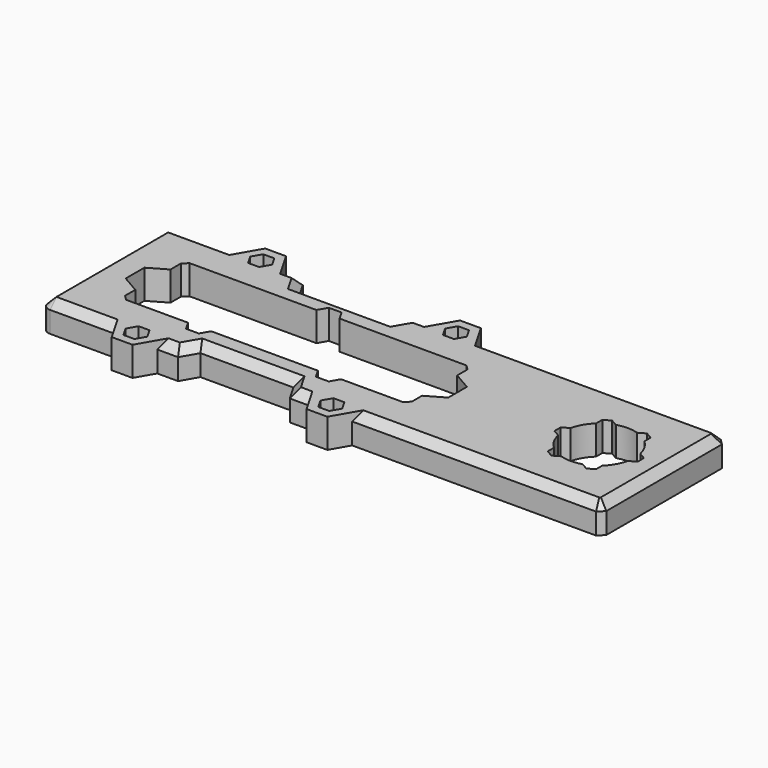
from build123d import *

# Parameters (mm, degrees)
F1_DEPTH      = 36.5
F2_SIZE       = 1.5
F4_DEPTH      = 75
F6_DEPTH      = 4.5
F8_DEPTH      = 4
F9_R          = 2.125
F10_DEPTH     = 4
F12_DEPTH     = 4
F13_R         = 2.125
F14_DEPTH     = 4
F15_R         = 2.125
F16_DEPTH     = 4
F18_DEPTH     = 32.75
F20_DEPTH     = 10
F21_R         = 2.125
F22_DEPTH     = 2
F23_W         = 33.9925625842
F23_H         = 3.75
F24_DEPTH     = 98.9435625842
F26_DEPTH     = 99
F27_T1_DEPTH  = 32.9343170514
F27_T3_DEPTH  = 25.8411991172
F28_T4_ANGLE  = 218.6312749598
F28_S5_R      = 11
F28_T6_DEPTH  = 16
F29_R         = 12.225
F29_R_2       = 4
F30_DEPTH     = 10
F31_T2_ANGLE  = 144.1325719132
F33_R         = 25
F34_DEPTH     = 25
F36_DEPTH     = 56.751
F37_T1_DEPTH  = 60.3629835333
F37_T3_DEPTH  = 29.9319647398
F37_T5_DEPTH  = 22.2894021556
F37_T7_DEPTH  = 111.8537479813
F37_T9_DEPTH  = 65.7902583728
F37_T11_DEPTH = 111.8554017465
F37_T13_DEPTH = 22.1084149398
F37_T15_DEPTH = 60.0584149398
F37_T17_DEPTH = 29.750977524
F40_DEPTH     = 56.751
F41_SIZE      = 1.5
F44_DEPTH     = 4
F45_R         = 2.125
F46_DEPTH     = 25
F47_R         = 2.125
F48_DEPTH     = 5
F50_DEPTH     = 4
F51_W         = 107.4425625842
F51_H         = 48
F52_DEPTH     = 47.751
F53_W         = 5
F53_H         = 48
F54_DEPTH     = 9
F55_R         = 2.5
F56_W         = 60
F56_H         = 48
F57_DEPTH     = 9
F58_SIZE      = 1.75
F59_W         = 4
F59_H         = 5.835
F60_DEPTH     = 9
F61_SIZE      = 2.49999


# Not quite as in the source:
# - a fillet or chamfer that OpenCascade refuses, or shapes differently, is made with other operations: its cross-section is extruded or revolved along the edge and cut away or added
# - a fillet or chamfer is up to 0.001 mm smaller than in the source, because OpenCascade refuses the exact size
# - after a boolean that leaves OpenCascade's solid faulty, fix() repairs it
# - a feature of the source that left no trace in its solid (it failed there, or was rolled back) is left out


with BuildPart() as f1:
    # F0 (on Top) → F1 (new body)
    with BuildSketch(Plane.XY):
        Polygon((-15.2700217866, -14.225), (0, -14.225), (15.2700217866, -14.225), (16.8700217866, -16.9962812921), (23.1299782134, -16.9962812921), (24.7299782134, -14.225), (46.15, -14.225), (46.15, -7.9299782134), (51.6925625842, -4.7299782134), (51.6925625842, 4.7299782134), (46.15, 7.9299782134), (46.15, 14.225), (4.7299782134, 14.225), (3.1299782134, 16.9962812921), (0, 16.9962812921), (-3.1299782134, 16.9962812921), (-4.7299782134, 14.225), (-46.15, 14.225), (-54.15, 14.225), (-54.15, -14.225), (-46.15, -14.225), (-24.7299782134, -14.225), (-23.1299782134, -16.9962812921), (-16.8700217866, -16.9962812921), align=None)
        Polygon((-1.975277675, 14.9962812921), (0, 14.9962812921), (1.975277675, 14.9962812921), (3.575277675, 12.225), (44.15, 12.225), (44.15, 6.775277675), (49.6925625842, 3.575277675), (49.6925625842, 0), (49.6925625842, -3.575277675), (44.15, -6.775277675), (44.15, -12.225), (23.575277675, -12.225), (21.975277675, -14.9962812921), (18.024722325, -14.9962812921), (16.424722325, -12.225), (3.575277675, -12.225), (-3.575277675, -12.225), (-16.424722325, -12.225), (-18.024722325, -14.9962812921), (-21.975277675, -14.9962812921), (-23.575277675, -12.225), (-44.15, -12.225), (-44.15, -6.775277675), (-49.6925625842, -3.575277675), (-49.6925625842, 0), (-49.6925625842, 3.575277675), (-44.15, 6.775277675), (-44.15, 12.225), (-3.575277675, 12.225), align=None, mode=Mode.SUBTRACT)
    extrude(amount=F1_DEPTH)

    # F2
    f2_edges = [f1.edges().sort_by_distance(p)[0] for p in [
        (-44.15, 12.225, 18.25),
        (44.15, 12.225, 18.25),
        (44.15, -12.225, 18.25),
        (-44.15, -12.225, 18.25),
    ]]
    chamfer(f2_edges, length=F2_SIZE)

    # F3 (on Right) → F4 (cut, symmetric)
    with BuildSketch(Plane.YZ):
        with BuildLine():
            Line((-11, 36.5), (-11, 32.75))
            ThreePointArc((-11, 32.75), (0, 21.75), (11, 32.75))
            Line((11, 32.75), (11, 36.5))
            Line((11, 36.5), (10.34105894, 36.5))
            ThreePointArc((10.34105894, 36.5), (0, 43.75), (-10.34105894, 36.5))
            Line((-10.34105894, 36.5), (-11, 36.5))
        make_face()
    extrude(amount=F4_DEPTH, both=True, mode=Mode.SUBTRACT)

    # F5 (on face) → F6 (join)
    with BuildSketch(Plane(origin=(-54.15, 0, 0), x_dir=(0, -1, 0), z_dir=(-1, 0, 0))):
        with BuildLine():
            Line((-24, 0), (-14.225, 0))
            Line((-14.225, 0), (14.225, 0))
            Line((14.225, 0), (24, 0))
            Line((24, 0), (24, 32.75))
            ThreePointArc((24, 32.75), (0, 56.75), (-24, 32.75))
            Line((-24, 32.75), (-24, 0))
        make_face()
        Polygon((-15.0825, 16.4344194104), (-15.0825, 13.0655805896), (-18, 11.3811611793), (-20.9175, 13.0655805896), (-20.9175, 16.4344194104), (-18, 18.1188388207), align=None, mode=Mode.SUBTRACT)
        Polygon((18, 18.1188388207), (20.9175, 16.4344194104), (20.9175, 13.0655805896), (18, 11.3811611793), (15.0825, 13.0655805896), (15.0825, 16.4344194104), align=None, mode=Mode.SUBTRACT)
        with BuildLine():
            ThreePointArc((-11, 32.75), (0, 43.75), (11, 32.75))
            ThreePointArc((11, 32.75), (0, 21.75), (-11, 32.75))
        make_face(mode=Mode.SUBTRACT)
        Polygon((0, 54.1188388207), (2.9175, 52.4344194104), (2.9175, 49.0655805896), (0, 47.3811611793), (-2.9175, 49.0655805896), (-2.9175, 52.4344194104), align=None, mode=Mode.SUBTRACT)
    extrude(amount=-F6_DEPTH)

    # F7 (on face) → F8 (join)
    with BuildSketch(Plane.YZ.offset(-49.65)):
        Polygon((-20.9175, 0), (-20.9175, 13.0655805896), (-20.9175, 16.4344194104), (-18, 18.1188388207), (-15.0825, 16.4344194104), (-15.0825, 13.0655805896), (-15.0825, 0), (-14.225, 0), (-14.225, 32.75), (-24, 32.75), (-24, 0), align=None)
        Polygon((20.9175, 16.4344194104), (20.9175, 13.0655805896), (20.9175, 0), (24, 0), (24, 32.75), (14.225, 32.75), (14.225, 0), (15.0825, 0), (15.0825, 13.0655805896), (15.0825, 16.4344194104), (18, 18.1188388207), align=None)
    extrude(amount=F8_DEPTH)

    # F9 (on face) → F10 (join)
    with BuildSketch(Plane(origin=(-54.15, 0, 0), x_dir=(0, -1, 0), z_dir=(-1, 0, 0))):
        Polygon((20.9175, 13.0655805896), (20.9175, 16.4344194104), (18, 18.1188388207), (15.0825, 16.4344194104), (15.0825, 13.0655805896), (15.0825, 0), (20.9175, 0), align=None)
        with Locations((18, 14.75)):
            Circle(F9_R, mode=Mode.SUBTRACT)
        Polygon((-15.0825, 16.4344194104), (-18, 18.1188388207), (-20.9175, 16.4344194104), (-20.9175, 13.0655805896), (-20.9175, 0), (-15.0825, 0), (-15.0825, 13.0655805896), align=None)
        with Locations((-18, 14.75)):
            Circle(F9_R, mode=Mode.SUBTRACT)
    extrude(amount=-F10_DEPTH)

    # F11 (on face) → F12 (join)
    with BuildSketch(Plane.YZ.offset(-49.65)):
        with BuildLine():
            Line((-24, 32.75), (-11, 32.75))
            ThreePointArc((-11, 32.75), (0, 43.75), (11, 32.75))
            Line((11, 32.75), (24, 32.75))
            ThreePointArc((24, 32.75), (17.9724789609, 48.6556593702), (2.9175, 56.5720106991))
            Line((2.9175, 56.5720106991), (2.9175, 52.4344194104))
            Line((2.9175, 52.4344194104), (2.9175, 49.0655805896))
            Line((2.9175, 49.0655805896), (0, 47.3811611793))
            Line((0, 47.3811611793), (-2.9175, 49.0655805896))
            Line((-2.9175, 49.0655805896), (-2.9175, 52.4344194104))
            Line((-2.9175, 52.4344194104), (-2.9175, 56.5720106991))
            ThreePointArc((-2.9175, 56.5720106991), (-17.9724789609, 48.6556593702), (-24, 32.75))
        make_face()
    extrude(amount=F12_DEPTH)

    # F13 (on face) → F14 (join)
    with BuildSketch(Plane(origin=(-54.15, 0, 0), x_dir=(0, -1, 0), z_dir=(-1, 0, 0))):
        Polygon((2.9175, 49.0655805896), (2.9175, 52.4344194104), (0, 54.1188388207), (-2.9175, 52.4344194104), (-2.9175, 49.0655805896), (0, 47.3811611793), align=None)
        with Locations((0, 50.75)):
            Circle(F13_R, mode=Mode.SUBTRACT)
    extrude(amount=-F14_DEPTH)

    # F15 (on face) → F16 (join)
    with BuildSketch(Plane.YZ.offset(-49.65)):
        Polygon((-20.9175, 16.4344194104), (-20.9175, 13.0655805896), (-18, 11.3811611793), (-15.0825, 13.0655805896), (-15.0825, 16.4344194104), (-18, 18.1188388207), align=None)
        with Locations((-18, 14.75)):
            Circle(F15_R, mode=Mode.SUBTRACT)
        Polygon((18, 11.3811611793), (20.9175, 13.0655805896), (20.9175, 16.4344194104), (18, 18.1188388207), (15.0825, 16.4344194104), (15.0825, 13.0655805896), align=None)
        with Locations((18, 14.75)):
            Circle(F15_R, mode=Mode.SUBTRACT)
    extrude(amount=-F16_DEPTH)

    # F17 (on Top) → F18 (join)
    with BuildSketch(Plane.XY):
        Polygon((-16.8700217866, -16.9962812921), (-23.1299782134, -16.9962812921), (-24.7299782134, -14.225), (-45.65, -14.225), (-45.65, -24), (-20.913620668, -24), (46.15, -24), (53.2925625842, -24), (53.2925625842, 24), (46.15, 24), (-20.913620668, 24), (-45.65, 24), (-45.65, 14.225), (-24.7299782134, 14.225), (-4.7299782134, 14.225), (-3.1299782134, 16.9962812921), (3.1299782134, 16.9962812921), (4.7299782134, 14.225), (46.15, 14.225), (46.15, 7.9299782134), (51.6925625842, 4.7299782134), (51.6925625842, -4.7299782134), (46.15, -7.9299782134), (46.15, -14.225), (24.7299782134, -14.225), (23.1299782134, -16.9962812921), (16.8700217866, -16.9962812921), (15.2700217866, -14.225), (-15.2700217866, -14.225), align=None)
    extrude(amount=F18_DEPTH)

    # F19 (on face) → F20 (cut)
    with BuildSketch(Plane.YZ.offset(53.2925625842)):
        with BuildLine():
            Line((11, 36.5), (10.34105894, 36.5))
            ThreePointArc((10.34105894, 36.5), (0, 43.75), (-10.34105894, 36.5))
            Line((-10.34105894, 36.5), (-11, 36.5))
            Line((-11, 36.5), (-11, 32.75))
            ThreePointArc((-11, 32.75), (0, 21.75), (11, 32.75))
            Line((11, 32.75), (11, 36.5))
        make_face()
    extrude(amount=-F20_DEPTH, mode=Mode.SUBTRACT)

    # F21 (on face) → F22 (join)
    with BuildSketch(Plane.YZ.offset(-49.65)):
        Polygon((2.9175, 49.0655805896), (2.9175, 52.4344194104), (0, 54.1188388207), (-2.9175, 52.4344194104), (-2.9175, 49.0655805896), (0, 47.3811611793), align=None)
        with Locations((0, 50.75)):
            Circle(F21_R, mode=Mode.SUBTRACT)
    extrude(amount=-F22_DEPTH)

    # F23 (on face) → F24 (cut, through all)
    with BuildSketch(Plane.YZ.offset(-45.65)):
        with Locations((0, 34.625)):
            Rectangle(F23_W, F23_H)
    extrude(amount=F24_DEPTH, mode=Mode.SUBTRACT)

    add(f1.part.fix(), mode=Mode.REPLACE)

    # F25 (on face) → F26 (join)
    with BuildSketch(Plane.YZ.offset(-45.65)):
        with BuildLine():
            ThreePointArc((-12.225, 32.75), (0, 44.975), (12.225, 32.75))
            Line((12.225, 32.75), (21.1201428428, 32.75))
            Line((21.1201428428, 32.75), (21.0697321738, 34.2564188517))
            Line((21.0697321738, 34.2564188517), (23.7859507749, 35.9482097699))
            ThreePointArc((23.7859507749, 35.9482097699), (22.1734543946, 41.9335679456), (19.0817785331, 47.3062951335))
            Line((19.0817785331, 47.3062951335), (15.990815889, 46.4780741892))
            Line((15.990815889, 46.4780741892), (13.7280741892, 48.740815889))
            Line((13.7280741892, 48.740815889), (14.5562951335, 51.8317785331))
            ThreePointArc((14.5562951335, 51.8317785331), (9.0526697354, 54.9772168897), (2.9175, 56.5720106991))
            Line((2.9175, 56.5720106991), (1.45875, 54.0453815836))
            Line((1.45875, 54.0453815836), (-1.45875, 54.0453815836))
            Line((-1.45875, 54.0453815836), (-2.9175, 56.5720106991))
            ThreePointArc((-2.9175, 56.5720106991), (-9.0526697354, 54.9772168897), (-14.5562951335, 51.8317785331))
            Line((-14.5562951335, 51.8317785331), (-13.7280741892, 48.740815889))
            Line((-13.7280741892, 48.740815889), (-15.990815889, 46.4780741892))
            Line((-15.990815889, 46.4780741892), (-19.0817785331, 47.3062951335))
            ThreePointArc((-19.0817785331, 47.3062951335), (-22.1734543946, 41.9335679456), (-23.7859507749, 35.9482097699))
            Line((-23.7859507749, 35.9482097699), (-21.0697321738, 34.2564188517))
            Line((-21.0697321738, 34.2564188517), (-21.1201428428, 32.75))
            Line((-21.1201428428, 32.75), (-12.225, 32.75))
        make_face()
    extrude(amount=F26_DEPTH)

    add(f1.part.fix(), mode=Mode.REPLACE)

    # F27: chamfer of 5 on 8 edges, made by hand

    # F27_s2 → F27_t1 (cut)
    with BuildSketch(Plane.YZ.offset(-16.4671585257)):
        with BuildLine():
            Line((17.225, 32.75), (11.2025051125, 37.6443338878))
            ThreePointArc((11.2025051125, 37.6443338878), (11.9500937859, 35.3279611147), (12.225, 32.75))
            Line((12.225, 32.75), (17.225, 32.75))
        make_face()
    extrude(amount=F27_T1_DEPTH, mode=Mode.SUBTRACT)

    # F27_s4 → F27_t3 (cut)
    with BuildSketch(Plane.YZ.offset(40.4006817335)):
        with BuildLine():
            Line((17.225, 32.75), (11.2025051125, 37.6443338878))
            ThreePointArc((11.2025051125, 37.6443338878), (11.9500937859, 35.3279611147), (12.225, 32.75))
            Line((12.225, 32.75), (17.225, 32.75))
        make_face()
    extrude(amount=F27_T3_DEPTH, mode=Mode.SUBTRACT)

    # F28: chamfer of 1.6 on 1 edges, made by hand


with BuildPart() as f28_tool2:
    # F28_s3 → F28_t4 (revolve)
    with BuildSketch(Plane(origin=(0, -10.2230123465, 29.1668194001), x_dir=(1, 0, 0), z_dir=(0, 0.3307719678, -0.9437107106))):
        Polygon((-44.05, 1.3922180559), (-45.65, -0.2077819441), (-45.65, 1.3922180559), align=None)
    revolve(axis=Axis((-45.65, 0, 32.75), (-1, 0, 0)), revolution_arc=F28_T4_ANGLE)

    # F28_s5 → F28_t6 (cut, symmetric)
    with BuildSketch(Plane.YZ.offset(-44.8)):
        with Locations((0, 32.75)):
            Circle(F28_S5_R)
    extrude(amount=F28_T6_DEPTH, both=True, mode=Mode.SUBTRACT)


with BuildPart() as f1_1:
    add(f1.part)

    # F28_t1: union F28_tool2
    add(f28_tool2.part)

    # F29 (on face) → F30 (join)
    with BuildSketch(Plane(origin=(44.15, 0, 0), x_dir=(0, -1, 0), z_dir=(-1, 0, 0))):
        with Locations((0, 32.75)):
            Circle(F29_R)
        with Locations((0, 32.75)):
            Circle(F29_R_2, mode=Mode.SUBTRACT)
    extrude(amount=-F30_DEPTH)

    # F31: chamfer of 5 on 2 edges, made by hand

    # F31_s1 → F31_t2 (revolve, cut)
    with BuildSketch(Plane(origin=(0, -3.4791810684, 0.3738774115), x_dir=(1, 0, 0), z_dir=(0, -0.9942755633, 0.1068461706))):
        Polygon((49.15, 44.787524699), (44.15, 39.787524699), (44.15, 44.787524699), align=None)
    revolve(axis=Axis((44.15, 0, 32.75), (-1, 0, 0)), revolution_arc=F31_T2_ANGLE, mode=Mode.SUBTRACT)

    # F33 (on face) → F34 (cut)
    with BuildSketch(Plane.YZ.offset(53.2925625842)):
        with Locations((0, 32.75)):
            Circle(F33_R)
    extrude(amount=F34_DEPTH, mode=Mode.SUBTRACT)

    # F35 (on Top) → F36 (cut, through all)
    with BuildSketch(Plane.XY):
        Polygon((-26.8, 29.5425625842), (-33.2, 29.5425625842), (-36.4, 24), (-33.2, 18.4574374158), (-26.8, 18.4574374158), (-23.6, 24), align=None)
        Polygon((33.2, 29.5425625842), (26.8, 29.5425625842), (23.6, 24), (26.8, 18.4574374158), (33.2, 18.4574374158), (36.4, 24), align=None)
        Polygon((33.2, -29.5425625842), (36.4, -24), (33.2, -18.4574374158), (26.8, -18.4574374158), (23.6, -24), (26.8, -29.5425625842), align=None)
        Polygon((-33.2, -29.5425625842), (-26.8, -29.5425625842), (-23.6, -24), (-26.8, -18.4574374158), (-33.2, -18.4574374158), (-36.4, -24), align=None)
    extrude(amount=F36_DEPTH, mode=Mode.SUBTRACT)

    # F37: chamfer of 2.5 on 18 edges, made by hand

    # F37_s2 → F37_t1 (cut)
    with BuildSketch(Plane.YZ.offset(-30.1814917667)):
        with BuildLine():
            Line((-23.3242090481, 38.4051986949), (-21.6639049928, 34.626498115))
            Line((-21.6639049928, 34.626498115), (-23.7859507749, 35.9482097699))
            ThreePointArc((-23.7859507749, 35.9482097699), (-23.5794343002, 37.2232849322), (-23.3242090481, 38.4051986949))
        make_face()
        with BuildLine():
            Line((23.3242090481, 38.4051986949), (21.6639049928, 34.626498115))
            Line((21.6639049928, 34.626498115), (23.7859507749, 35.9482097699))
            ThreePointArc((23.7859507749, 35.9482097699), (23.5794343002, 37.2232849322), (23.3242090481, 38.4051986949))
        make_face()
    extrude(amount=F37_T1_DEPTH, mode=Mode.SUBTRACT)

    # F37_s4 → F37_t3 (cut)
    with BuildSketch(Plane.YZ.offset(29.8185082333)):
        with BuildLine():
            Line((-23.3242090481, 38.4051986949), (-21.6639049928, 34.626498115))
            Line((-21.6639049928, 34.626498115), (-23.7859507749, 35.9482097699))
            ThreePointArc((-23.7859507749, 35.9482097699), (-23.5794343002, 37.2232849322), (-23.3242090481, 38.4051986949))
        make_face()
        with BuildLine():
            Line((23.3242090481, 38.4051986949), (21.6639049928, 34.626498115))
            Line((21.6639049928, 34.626498115), (23.7859507749, 35.9482097699))
            ThreePointArc((23.7859507749, 35.9482097699), (23.5794343002, 37.2232849322), (23.3242090481, 38.4051986949))
        make_face()
    extrude(amount=F37_T3_DEPTH, mode=Mode.SUBTRACT)

    # F37_s6 → F37_t5 (cut)
    with BuildSketch(Plane.YZ.offset(-52.1079103889)):
        with BuildLine():
            Line((-23.3242090481, 38.4051986949), (-21.6639049928, 34.626498115))
            Line((-21.6639049928, 34.626498115), (-23.7859507749, 35.9482097699))
            ThreePointArc((-23.7859507749, 35.9482097699), (-23.5794343002, 37.2232849322), (-23.3242090481, 38.4051986949))
        make_face()
        with BuildLine():
            Line((23.3242090481, 38.4051986949), (21.6639049928, 34.626498115))
            Line((21.6639049928, 34.626498115), (23.7859507749, 35.9482097699))
            ThreePointArc((23.7859507749, 35.9482097699), (23.5794343002, 37.2232849322), (23.3242090481, 38.4051986949))
        make_face()
    extrude(amount=F37_T5_DEPTH, mode=Mode.SUBTRACT)

    # F37_s8 → F37_t7 (cut)
    with BuildSketch(Plane.YZ.offset(-52.1055926985)):
        with BuildLine():
            Line((-13.9092475207, 49.4169639674), (-12.4923347158, 53.242476018))
            ThreePointArc((-12.4923347158, 53.242476018), (-13.5089916223, 52.5870145271), (-14.5562951335, 51.8317785331))
            Line((-14.5562951335, 51.8317785331), (-13.9092475207, 49.4169639674))
        make_face()
        with BuildLine():
            Line((12.4923347158, 53.242476018), (13.9092475207, 49.4169639674))
            Line((13.9092475207, 49.4169639674), (14.5562951335, 51.8317785331))
            ThreePointArc((14.5562951335, 51.8317785331), (13.5089916223, 52.5870145271), (12.4923347158, 53.242476018))
        make_face()
    extrude(amount=F37_T7_DEPTH, mode=Mode.SUBTRACT)

    # F37_s10 → F37_t9 (cut)
    with BuildSketch(Plane.YZ.offset(-32.8951291864)):
        with BuildLine():
            Line((-16.6669639674, 46.6592475207), (-20.492476018, 45.2423347158))
            ThreePointArc((-20.492476018, 45.2423347158), (-19.8370145271, 46.2589916223), (-19.0817785331, 47.3062951335))
            Line((-19.0817785331, 47.3062951335), (-16.6669639674, 46.6592475207))
        make_face()
        with BuildLine():
            Line((16.6669639674, 46.6592475207), (20.492476018, 45.2423347158))
            ThreePointArc((20.492476018, 45.2423347158), (19.8370145271, 46.2589916223), (19.0817785331, 47.3062951335))
            Line((19.0817785331, 47.3062951335), (16.6669639674, 46.6592475207))
        make_face()
    extrude(amount=F37_T9_DEPTH, mode=Mode.SUBTRACT)

    # F37_s12 → F37_t11 (cut)
    with BuildSketch(Plane.YZ.offset(-52.1064195811)):
        with BuildLine():
            Line((-5.3797630169, 56.1392742487), (-1.6675, 54.4069471897))
            Line((-1.6675, 54.4069471897), (-2.9175, 56.5720106991))
            ThreePointArc((-2.9175, 56.5720106991), (-4.1946176733, 56.3805984388), (-5.3797630169, 56.1392742487))
        make_face()
        with BuildLine():
            Line((1.6675, 54.4069471897), (5.3797630169, 56.1392742487))
            ThreePointArc((5.3797630169, 56.1392742487), (4.1946176733, 56.3805984388), (2.9175, 56.5720106991))
            Line((2.9175, 56.5720106991), (1.6675, 54.4069471897))
        make_face()
    extrude(amount=F37_T11_DEPTH, mode=Mode.SUBTRACT)

    # F37_s14 → F37_t13 (cut)
    with BuildSketch(Plane.YZ.offset(-52.0792074699)):
        Polygon((-24, 30.25), (-21.5, 32.75), (-24, 32.75), align=None)
        Polygon((24, 30.25), (21.5, 32.75), (24, 32.75), align=None)
    extrude(amount=F37_T13_DEPTH, mode=Mode.SUBTRACT)

    # F37_s16 → F37_t15 (cut)
    with BuildSketch(Plane.YZ.offset(-30.0292074699)):
        Polygon((-21.5, 32.75), (-24, 30.25), (-24, 32.75), align=None)
        Polygon((24, 30.25), (21.5, 32.75), (24, 32.75), align=None)
    extrude(amount=F37_T15_DEPTH, mode=Mode.SUBTRACT)

    # F37_s18 → F37_t17 (cut)
    with BuildSketch(Plane.YZ.offset(29.9707925301)):
        Polygon((-21.5, 32.75), (-24, 30.25), (-24, 32.75), align=None)
        Polygon((21.5, 32.75), (24, 30.25), (24, 32.75), align=None)
    extrude(amount=F37_T17_DEPTH, mode=Mode.SUBTRACT)

    # F39 (on Top) → F40 (cut, through all)
    with BuildSketch(Plane.XY):
        Polygon((-17.2, -24), (0, -24), (17.2, -24), (14.3132486541, -19), (0, -19), (-14.3132486541, -19), align=None)
        Polygon((17.2, 24), (0, 24), (-17.2, 24), (-14.3132486541, 19), (0, 19), (14.3132486541, 19), align=None)
    extrude(amount=F40_DEPTH, mode=Mode.SUBTRACT)

    # F41
    f41_edges = [f1_1.edges().sort_by_distance(p)[0] for p in [
        (0, -19, 45.795126),
        (29.847565, -18.457437, 45.996083),
        (-29.847565, -18.457437, 45.996083),
        (0, 19, 45.795126),
        (29.847565, 18.457437, 45.996083),
        (-29.847565, 18.457437, 45.996083),
    ]]
    chamfer(f41_edges, length=F41_SIZE)

    # F43 (on offset) → F44 (cut)
    with BuildSketch(Plane.YZ.offset(47)):
        Polygon((2.9175, 44.3155805896), (2.9175, 47.6844194104), (2.9175, 59.0453815836), (0, 59.0453815836), (-2.9175, 59.0453815836), (-2.9175, 47.6844194104), (-2.9175, 44.3155805896), (0, 42.6311611793), align=None)
        Polygon((-12.0825, 13.3155805896), (-12.0825, 16.6844194104), (-15, 18.3688388207), (-17.9175, 16.6844194104), (-17.9175, 13.3155805896), (-17.9175, 0), (-12.0825, 0), align=None)
        Polygon((15, 18.3688388207), (12.0825, 16.6844194104), (12.0825, 13.3155805896), (12.0825, 0), (17.9175, 0), (17.9175, 13.3155805896), (17.9175, 16.6844194104), align=None)
    extrude(amount=F44_DEPTH, mode=Mode.SUBTRACT)

    # F45 (on offset) → F46 (cut)
    with BuildSketch(Plane.YZ.offset(47)):
        with Locations((-15, 15)):
            Circle(F45_R)
        with Locations((0, 46)):
            Circle(F45_R)
        with Locations((15, 15)):
            Circle(F45_R)
    extrude(amount=F46_DEPTH, mode=Mode.SUBTRACT)

    # F47 (on Top) → F48 (join)
    with BuildSketch(Plane.XY):
        Polygon((-26.8, 29.5425625842), (-33.2, 29.5425625842), (-36.4, 24), (-33.2, 18.4574374158), (-26.8, 18.4574374158), (-23.6, 24), align=None)
        with Locations((-30, 24)):
            Circle(F47_R, mode=Mode.SUBTRACT)
        Polygon((23.6, 24), (26.8, 18.4574374158), (33.2, 18.4574374158), (36.4, 24), (33.2, 29.5425625842), (26.8, 29.5425625842), align=None)
        with Locations((30, 24)):
            Circle(F47_R, mode=Mode.SUBTRACT)
        Polygon((36.4, -24), (33.2, -18.4574374158), (26.8, -18.4574374158), (23.6, -24), (26.8, -29.5425625842), (33.2, -29.5425625842), align=None)
        with Locations((30, -24)):
            Circle(F47_R, mode=Mode.SUBTRACT)
        Polygon((-36.4, -24), (-33.2, -29.5425625842), (-26.8, -29.5425625842), (-23.6, -24), (-26.8, -18.4574374158), (-33.2, -18.4574374158), align=None)
        with Locations((-30, -24)):
            Circle(F47_R, mode=Mode.SUBTRACT)
    extrude(amount=F48_DEPTH)

    # F49 (on face) → F50 (join)
    with BuildSketch(Plane.XY.offset(5)):
        Polygon((-26.8, -18.4574374158), (-33.2, -18.4574374158), (-36.4, -24), (-33.2, -29.5425625842), (-26.8, -29.5425625842), (-23.6, -24), align=None)
        Polygon((-33.3688388207, -24), (-31.6844194104, -21.0825), (-28.3155805896, -21.0825), (-26.6311611793, -24), (-28.3155805896, -26.9175), (-31.6844194104, -26.9175), align=None, mode=Mode.SUBTRACT)
        Polygon((23.6, -24), (26.8, -29.5425625842), (33.2, -29.5425625842), (36.4, -24), (33.2, -18.4574374158), (26.8, -18.4574374158), align=None)
        Polygon((28.3155805896, -21.0825), (31.6844194104, -21.0825), (33.3688388207, -24), (31.6844194104, -26.9175), (28.3155805896, -26.9175), (26.6311611793, -24), align=None, mode=Mode.SUBTRACT)
        Polygon((26.8, 29.5425625842), (23.6, 24), (26.8, 18.4574374158), (33.2, 18.4574374158), (36.4, 24), (33.2, 29.5425625842), align=None)
        Polygon((31.6844194104, 21.0825), (28.3155805896, 21.0825), (26.6311611793, 24), (28.3155805896, 26.9175), (31.6844194104, 26.9175), (33.3688388207, 24), align=None, mode=Mode.SUBTRACT)
        Polygon((-36.4, 24), (-33.2, 18.4574374158), (-26.8, 18.4574374158), (-23.6, 24), (-26.8, 29.5425625842), (-33.2, 29.5425625842), align=None)
        Polygon((-31.6844194104, 26.9175), (-28.3155805896, 26.9175), (-26.6311611793, 24), (-28.3155805896, 21.0825), (-31.6844194104, 21.0825), (-33.3688388207, 24), align=None, mode=Mode.SUBTRACT)
    extrude(amount=F50_DEPTH)

    # F51 (on face) → F52 (cut, through all)
    with BuildSketch(Plane.XY.offset(9)):
        with Locations((-0.4287187079, 0)):
            Rectangle(F51_W, F51_H)
    extrude(amount=F52_DEPTH, mode=Mode.SUBTRACT)

    # F53 (on Top) → F54 (join)
    with BuildSketch(Plane.XY):
        with Locations((-56.65, 0)):
            Rectangle(F53_W, F53_H)
    extrude(amount=F54_DEPTH)

    # F55
    f55_edges = [f1_1.edges().sort_by_distance(p)[0] for p in [
        (-59.15, -24, 4.5),
        (-59.15, 24, 4.5),
    ]]
    fillet(f55_edges, radius=F55_R)

    # F56 (on Top) → F57 (join)
    with BuildSketch(Plane.XY):
        with Locations((83.2925625842, 0)):
            Rectangle(F56_W, F56_H)
        with BuildLine():
            ThreePointArc((90.0035287932, 10.4967736339), (93.2925625842, 11), (96.5815963753, 10.4967736339))
            Line((96.5815963753, 10.4967736339), (98.6600573443, 11.6967736339))
            Line((98.6600573443, 11.6967736339), (100.7385183134, 10.4967736339))
            Line((100.7385183134, 10.4967736339), (100.7385183134, 8.0967736339))
            ThreePointArc((100.7385183134, 8.0967736339), (102.8188420258, 5.5), (104.0275521045, 2.4))
            Line((104.0275521045, 2.4), (106.1060130736, 1.2))
            Line((106.1060130736, 1.2), (106.1060130736, -1.2))
            Line((106.1060130736, -1.2), (104.0275521045, -2.4))
            ThreePointArc((104.0275521045, -2.4), (102.8188420258, -5.5), (100.7385183134, -8.0967736339))
            Line((100.7385183134, -8.0967736339), (100.7385183134, -10.4967736339))
            Line((100.7385183134, -10.4967736339), (98.6600573443, -11.6967736339))
            Line((98.6600573443, -11.6967736339), (96.5815963753, -10.4967736339))
            ThreePointArc((96.5815963753, -10.4967736339), (93.2925625842, -11), (90.0035287932, -10.4967736339))
            Line((90.0035287932, -10.4967736339), (87.9250678241, -11.6967736339))
            Line((87.9250678241, -11.6967736339), (85.846606855, -10.4967736339))
            Line((85.846606855, -10.4967736339), (85.846606855, -8.0967736339))
            ThreePointArc((85.846606855, -8.0967736339), (83.7662831426, -5.5), (82.557573064, -2.4))
            Line((82.557573064, -2.4), (80.4791120949, -1.2))
            Line((80.4791120949, -1.2), (80.4791120949, 1.2))
            Line((80.4791120949, 1.2), (82.557573064, 2.4))
            ThreePointArc((82.557573064, 2.4), (83.7662831426, 5.5), (85.846606855, 8.0967736339))
            Line((85.846606855, 8.0967736339), (85.846606855, 10.4967736339))
            Line((85.846606855, 10.4967736339), (87.9250678241, 11.6967736339))
            Line((87.9250678241, 11.6967736339), (90.0035287932, 10.4967736339))
        make_face(mode=Mode.SUBTRACT)
    extrude(amount=F57_DEPTH)

    # F58
    f58_edges = [f1_1.edges().sort_by_distance(p)[0] for p in [
        (113.292563, -24, 4.5),
        (113.292563, 24, 4.5),
    ]]
    chamfer(f58_edges, length=F58_SIZE)

    # F59 (on Top) → F60 (join)
    with BuildSketch(Plane.XY):
        with Locations((-47.65, 18)):
            Rectangle(F59_W, F59_H)
        with Locations((-47.65, -18)):
            Rectangle(F59_W, F59_H)
        with Locations((49, 15)):
            Rectangle(F59_W, F59_H)
        with Locations((49, -15)):
            Rectangle(F59_W, F59_H)
    extrude(amount=F60_DEPTH)

    # F61 (size 2.5 in the source; OpenCascade refuses exactly that, so slightly less here)
    f61_edges = [f1_1.edges().sort_by_distance(p)[0] for p in [
        (-46.525, 24, 9),
        (-59.15, 0, 9),
        (-46.525, -24, 9),
        (-58.417767, 23.267767, 9),
        (-20.4, -24, 9),
        (-15.756624, -21.5, 9),
        (0, -19, 9),
        (15.756624, -21.5, 9),
        (20.4, -24, 9),
        (-20.4, 24, 9),
        (-15.756624, 21.5, 9),
        (0, 19, 9),
        (15.756624, 21.5, 9),
        (20.4, 24, 9),
        (73.971281, 24, 9),
        (113.292563, 0, 9),
        (73.971281, -24, 9),
        (112.417563, 23.125, 9),
        (112.417563, -23.125, 9),
        (-58.417767, -23.267767, 9),
    ]]
    chamfer(f61_edges, length=F61_SIZE)


solid = f1_1.part
